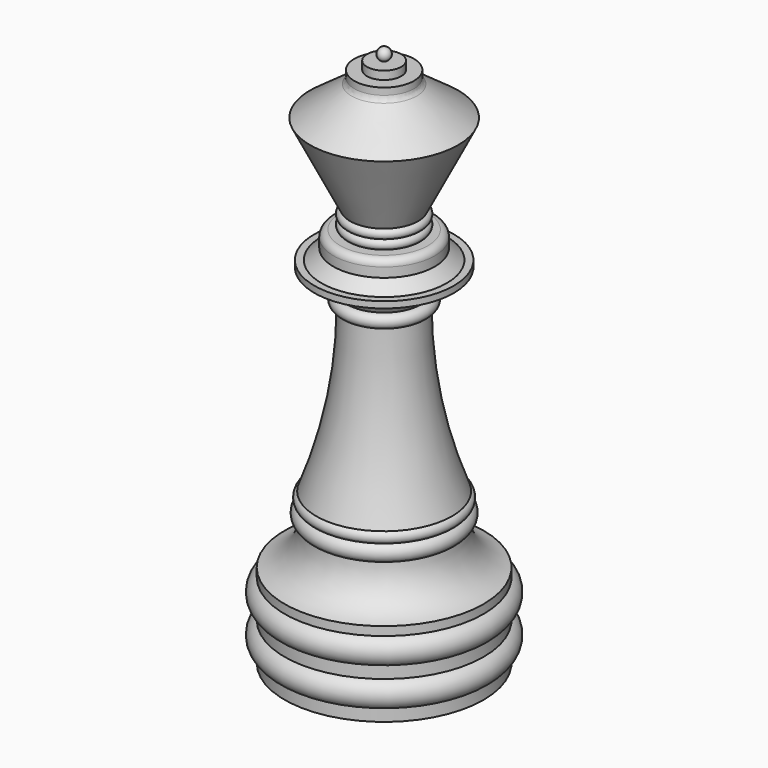
from build123d import *

# Parameters (mm, degrees)
F5_R     = 1
F6_R     = 1
F7_R     = 13.5
F8_DEPTH = 2
F9_R     = 1.99999


# Not quite as in the source:
# - a fillet or chamfer that OpenCascade refuses, or shapes differently, is made with other operations: its cross-section is extruded or revolved along the edge and cut away or added
# - a fillet or chamfer is up to 0.001 mm smaller than in the source, because OpenCascade refuses the exact size


with BuildPart() as f1:
    # F0 (on Front) → F1 (revolve)
    with BuildSketch(Plane.XZ):
        with BuildLine():
            Line((-203.3652514219, 101.259062287), (-203.3652514219, 22.761361911))
            Line((-203.3652514219, 22.761361911), (-188.6436624619, 22.761361911))
            Line((-188.6436624619, 22.761361911), (-188.6436624619, 24.5533513417))
            ThreePointArc((-188.6436624619, 24.5533513417), (-187.3838848671, 26.4532041654), (-188.6436624619, 28.3530569891))
            Line((-188.6436624619, 28.3530569891), (-188.6436624619, 30.1450464199))
            Line((-188.6436624619, 30.1450464199), (-188.6436624619, 33.9447520673))
            Line((-188.6436624619, 33.9447520673), (-188.6436624619, 35.2401472628))
            Line((-188.6436624619, 35.2401472628), (-193.309366703, 35.2401472628))
            Line((-193.309366703, 35.2401472628), (-193.309366703, 41.1680191755))
            ThreePointArc((-193.309366703, 41.1680191755), (-192.5565818681, 42.3696450889), (-193.309366703, 43.5712710023))
            ThreePointArc((-193.309366703, 43.5712710023), (-192.8404048548, 44.3696901202), (-193.309366703, 45.1681092381))
            Line((-193.309366703, 45.1681092381), (-197.8608220816, 45.1681092381))
            Line((-197.8608220816, 45.1681092381), (-197.8608220816, 69.3112561437))
            ThreePointArc((-197.8608220816, 69.3112561437), (-196.8800943317, 70.2974423766), (-197.8608220816, 71.2836286096))
            Line((-197.8608220816, 71.2836286096), (-197.8608220816, 74.3284672499))
            Line((-197.8608220816, 74.3284672499), (-193.0439472198, 74.3284672499))
            Line((-193.0439472198, 74.3284672499), (-193.0439472198, 75.2748303938))
            Line((-193.0439472198, 75.2748303938), (-194.0847486258, 75.2748303938))
            Line((-194.0847486258, 75.2748303938), (-195.8655714989, 76.8517457771))
            Line((-195.8655714989, 76.8517457771), (-195.8655714989, 79.2579033303))
            Line((-195.8655714989, 79.2579033303), (-198.3242481947, 79.2579033303))
            ThreePointArc((-198.3242481947, 79.2579033303), (-197.7911045704, 79.9374569619), (-198.3242481947, 80.6170105934))
            ThreePointArc((-198.3242481947, 80.6170105934), (-197.7911045704, 81.296564225), (-198.3242481947, 81.9761178565))
            Line((-198.3242481947, 81.9761178565), (-192.4043744802, 93.8070736003))
            Line((-192.4043744802, 93.8070736003), (-198.949098587, 98.5011926961))
            Line((-198.949098587, 98.5011926961), (-198.949098587, 100.0382101504))
            Line((-198.949098587, 100.0382101504), (-200.8288223515, 100.0382101504))
            Line((-200.8288223515, 100.0382101504), (-200.8288223515, 101.259062287))
            Line((-200.8288223515, 101.259062287), (-203.1206665266, 101.259062287))
            ThreePointArc((-203.1206665266, 101.259062287), (-202.4737595632, 102.2486501568), (-203.3652514219, 103.0251905853))
            Line((-203.3652514219, 103.0251905853), (-203.3652514219, 101.259062287))
        make_face()
        with BuildLine():
            Line((-188.6436624619, 33.9447520673), (-188.6436624619, 30.1450464199))
            ThreePointArc((-188.6436624619, 30.1450464199), (-187.3838848671, 32.0448992436), (-188.6436624619, 33.9447520673))
        make_face()
    revolve(axis=Axis((-203.3652514219, 0, 62.010212099), (0, 0, -1)))

    # F2: fillet of radius 6 on 1 edges, made by hand

    # F2_s1 → F2_t2 (revolve)
    with BuildSketch(Plane.XZ):
        with BuildLine():
            ThreePointArc((-188.6436624619, 35.2401472628), (-192.0000902375, 37.3486325423), (-193.309366703, 41.0899040806))
            Line((-193.309366703, 41.0899040806), (-193.429366703, 41.0899040806))
            Line((-193.429366703, 41.0899040806), (-193.429366703, 35.2401472628))
            Line((-193.429366703, 35.2401472628), (-193.309366703, 35.1201472628))
            ThreePointArc((-193.309366703, 35.1201472628), (-190.9765145825, 35.1201472628), (-188.6703483771, 35.1231521265))
            Line((-188.6703483771, 35.1231521265), (-188.6436624619, 35.2401472628))
        make_face()
    revolve(axis=Axis((-203.3652514219, 0, 35.2401472628), (0, 0, -1)))

    # F3: fillet of radius 66.3 on 1 edges, made by hand

    # F3_s1 → F3_t2 (revolve)
    with BuildSketch(Plane.XZ):
        with BuildLine():
            ThreePointArc((-197.8608220816, 69.3095101323), (-196.7130227674, 57.0261577479), (-193.309366703, 45.1681092381))
            Line((-193.309366703, 45.1681092381), (-194.5443375955, 44.6852812203))
            ThreePointArc((-194.5443375955, 44.6852812203), (-195.5850943923, 43.8421092381), (-197.8608220816, 43.8421092381))
            Line((-197.8608220816, 43.8421092381), (-199.1868220816, 45.1681092381))
            Line((-199.1868220816, 45.1681092381), (-199.1868220816, 69.3095101323))
            Line((-199.1868220816, 69.3095101323), (-197.8608220816, 69.3095101323))
        make_face()
    revolve(axis=Axis((-203.3652514219, 0, 45.1681092381), (0, 0, -1)))

    # F4: fillet of radius 5.33 on 1 edges, made by hand

    # F4_s1 → F4_t2 (revolve)
    with BuildSketch(Plane.XZ):
        with BuildLine():
            ThreePointArc((-193.0455404117, 74.3284672499), (-195.8941356754, 73.5033984395), (-197.8608220816, 71.2836286096))
            Line((-197.8608220816, 71.2836286096), (-197.957127715, 71.3293318368))
            ThreePointArc((-197.957127715, 71.3293318368), (-197.9674220816, 72.8060479297), (-197.9674220816, 74.3284672499))
            Line((-197.9674220816, 74.3284672499), (-197.8608220816, 74.4350672499))
            Line((-197.8608220816, 74.4350672499), (-193.0455404117, 74.4350672499))
            Line((-193.0455404117, 74.4350672499), (-193.0455404117, 74.3284672499))
        make_face()
    revolve(axis=Axis((-203.3652514219, 0, 74.3284672499), (0, 0, -1)))

    # F5
    f5_edges = [f1.edges().sort_by_distance(p)[0] for p in [
        (-210.864931, 0, 79.257903),
    ]]
    fillet(f5_edges, radius=F5_R)

    # F6
    f6_edges = [f1.edges().sort_by_distance(p)[0] for p in [
        (-207.781404, 0, 98.501193),
    ]]
    fillet(f6_edges, radius=F6_R)

    # F7 (on face) → F8 (cut)
    with BuildSketch(Plane(origin=(0, 0, 22.761361911), x_dir=(1, 0, 0), z_dir=(0, 0, -1))):
        with Locations((-203.3652514219, 0)):
            Circle(F7_R)
    extrude(amount=-F8_DEPTH, mode=Mode.SUBTRACT)

    # F9 (radius 2 in the source; OpenCascade refuses exactly that, so slightly less here)
    f9_edges = [f1.edges().sort_by_distance(p)[0] for p in [
        (-216.865251, 0, 24.761362),
    ]]
    fillet(f9_edges, radius=F9_R)


solid = f1.part
